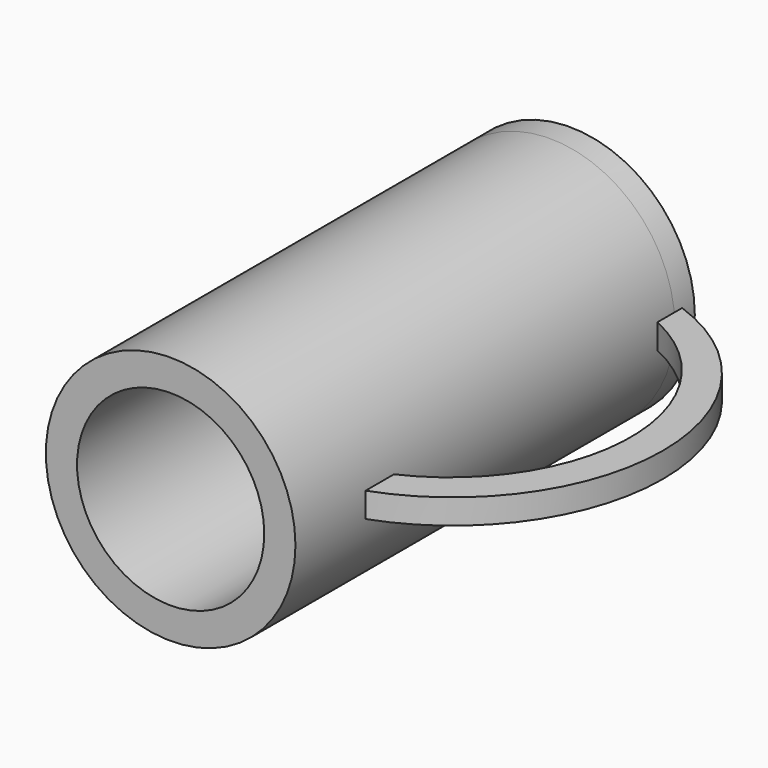
from build123d import *

# Parameters (mm, degrees)
F0_R     = 25.4
F0_R_2   = 19.05
F1_DEPTH = 101.6
F3_DEPTH = 2.54
F4_R     = 25.4
F5_DEPTH = 5.08


with BuildPart() as f1:
    # F0 (on Front) → F1 (new body)
    with BuildSketch(Plane.XZ):
        Circle(F0_R)
        Circle(F0_R_2, mode=Mode.SUBTRACT)
    extrude(amount=F1_DEPTH)


with BuildPart() as f3:
    # F2 (on Top) → F3 (new body, symmetric)
    with BuildSketch(Plane.XY):
        with BuildLine():
            Line((25.4, -76.5425107099), (25.4, -83.7568040209))
            ThreePointArc((25.4, -83.7568040209), (53.7095561275, -43.4922314016), (25.4, -3.2276587823))
            Line((25.4, -3.2276587823), (25.4, -9.4887303788))
            ThreePointArc((25.4, -9.4887303788), (46.8062490865, -43.0156205443), (25.4, -76.5425107099))
        make_face()
    extrude(amount=F3_DEPTH, both=True)


with BuildPart() as f5:
    # F4 (on Front) → F5 (new body)
    with BuildSketch(Plane.XZ):
        Circle(F4_R)
    extrude(amount=F5_DEPTH)


solid = Compound([f1.part, f3.part, f5.part])
